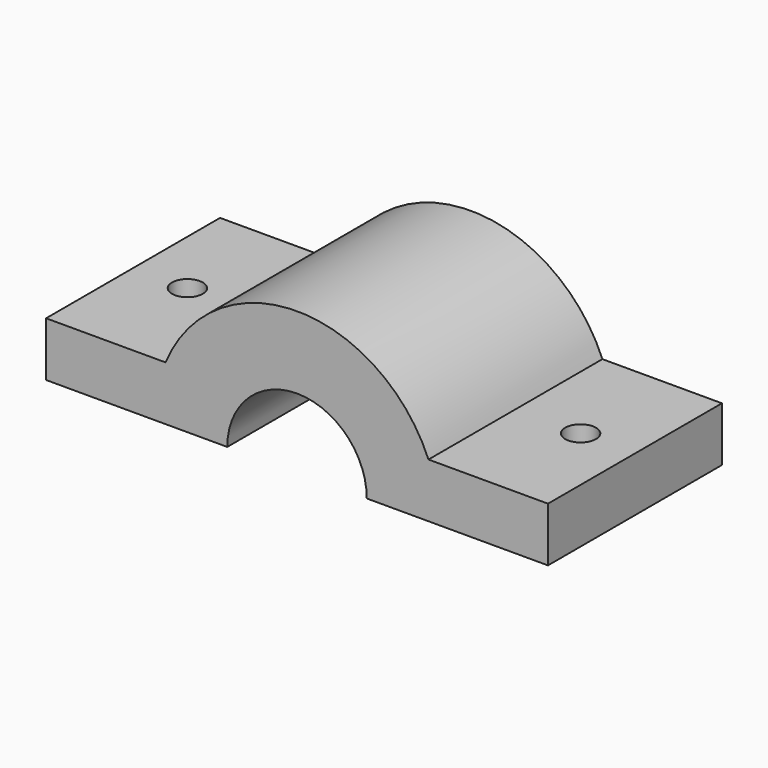
from build123d import *

# Parameters (mm, degrees)
F1_DEPTH = 24
F2_R     = 1.7
F3_DEPTH = 25


# Not quite as in the source:
# - a feature names something its author has since deleted; it is built from what else it names


with BuildPart() as f1:
    # F0 (on Front) → F1 (new body)
    with BuildSketch(Plane.XZ):
        with BuildLine():
            ThreePointArc((-7.7, 0), (0, 7.7), (7.7, 0))
            Line((7.7, 0), (15.7, 0))
            Line((15.7, 0), (27.7, 0))
            Line((27.7, 0), (27.7, 6))
            Line((27.7, 6), (14.5082735017, 6))
            ThreePointArc((14.5082735017, 6), (0, 15.7), (-14.5082735017, 6))
            Line((-14.5082735017, 6), (-27.7, 6))
            Line((-27.7, 6), (-27.7, 0))
            Line((-27.7, 0), (-15.7, 0))
            Line((-15.7, 0), (-7.7, 0))
        make_face()
    extrude(amount=F1_DEPTH)

    # F2 (on face) → F3 (cut)
    with BuildSketch(Plane.XY.offset(6)):
        with Locations((-21.7, -12)):
            Circle(F2_R)
        with Locations((21.7, -12)):
            Circle(F2_R)
    extrude(amount=-F3_DEPTH, mode=Mode.SUBTRACT)


solid = f1.part
